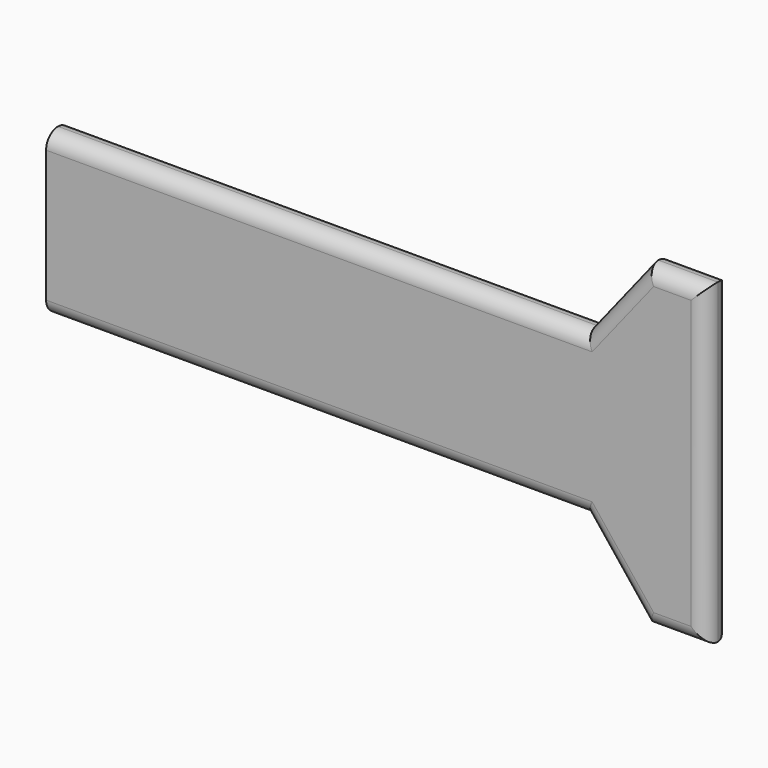
from build123d import *

# Parameters (mm, degrees)
F0_W     = 69.1453650223
F0_H     = 11.3406319083
F0_H_2   = 9.4049024593
F1_DEPTH = 3.81
F2_R     = 1.90499


# Not quite as in the source:
# - a fillet or chamfer is up to 0.001 mm smaller than in the source, because OpenCascade refuses the exact size


with BuildPart() as f1:
    # F0 (on Front) → F1 (new body)
    with BuildSketch(Plane.XZ):
        Polygon((46.6354282098, 21.2878647245), (38.7396977623, 11.3406319083), (38.7396977623, 0), (38.7396977623, -9.4049024593), (46.6354282098, -19.3521352755), (54.2554282098, -19.3521352755), (54.2554282098, 21.2878647245), align=None)
        with Locations((4.1670152511, 5.6703159541)):
            Rectangle(F0_W, F0_H)
        with Locations((4.1670152511, -4.7024512296)):
            Rectangle(F0_W, F0_H_2)
    extrude(amount=F1_DEPTH)

    # F2 (radius 1.905 in the source; OpenCascade refuses exactly that, so slightly less here)
    f2_edges = [f1.edges().sort_by_distance(p)[0] for p in [
        (4.167015, 0, -9.404902),
        (4.167015, 0, 11.340632),
        (4.167015, -3.81, -9.404902),
        (4.167015, -3.81, 11.340632),
        (50.445428, -3.81, -19.352135),
        (50.445428, 0, -19.352135),
        (50.445428, 0, 21.287865),
        (50.445428, -3.81, 21.287865),
        (54.255428, -3.81, 0.967865),
        (54.255428, 0, 0.967865),
        (42.687563, -3.81, 16.314248),
        (42.687563, -3.81, -14.378519),
        (42.687563, 0, -14.378519),
        (42.687563, 0, 16.314248),
    ]]
    fillet(f2_edges, radius=F2_R)


solid = f1.part
